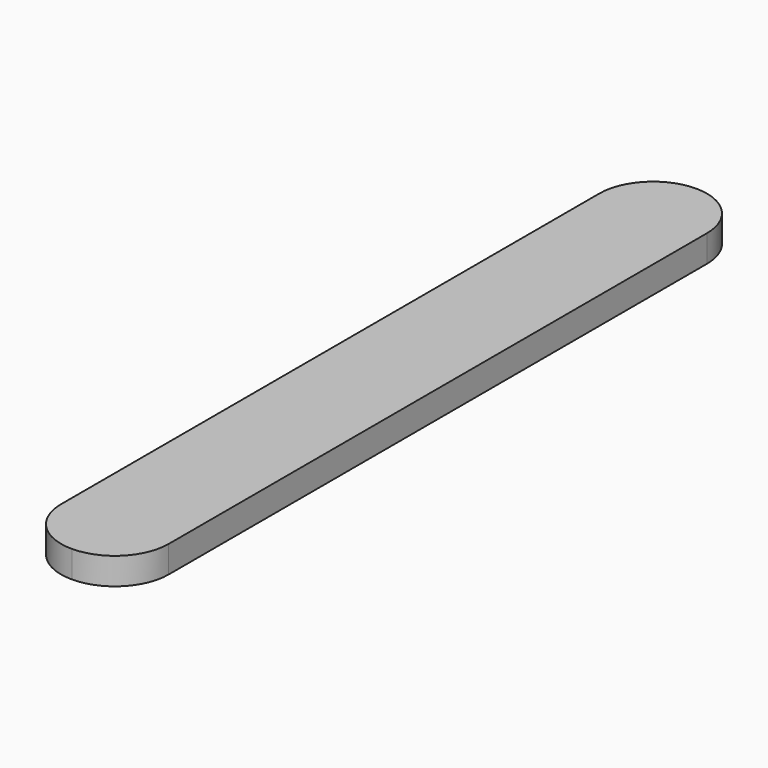
from build123d import *

# Parameters (mm, degrees)
F0_W     = 10
F0_H     = 72.5174620748
F1_DEPTH = 2.5
F2_R     = 4.99999


# Not quite as in the source:
# - a fillet or chamfer is up to 0.001 mm smaller than in the source, because OpenCascade refuses the exact size


with BuildPart() as f1:
    # F0 (on Top) → F1 (new body)
    with BuildSketch(Plane.XY):
        Rectangle(F0_W, F0_H)
    extrude(amount=F1_DEPTH)

    # F2 (radius 5 in the source; OpenCascade refuses exactly that, so slightly less here)
    f2_edges = [f1.edges().sort_by_distance(p)[0] for p in [
        (5, 36.258731, 1.25),
        (-5, 36.258731, 1.25),
        (-5, -36.258731, 1.25),
        (5, -36.258731, 1.25),
    ]]
    fillet(f2_edges, radius=F2_R)


solid = f1.part
